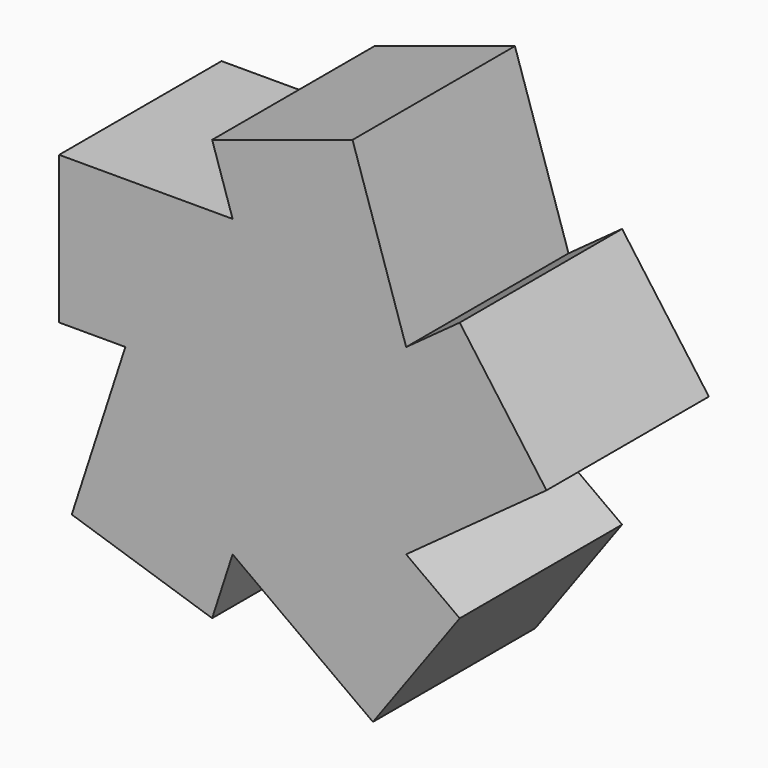
from build123d import *

# Parameters (mm, degrees)
F0_W     = 60
F0_H     = 55
F1_DEPTH = 40
F2_COUNT = 5


with BuildPart() as f1:
    # F0 (on Top) → F1 (new body)
    with BuildSketch(Plane.XY):
        with Locations((-30, 27.5)):
            Rectangle(F0_W, F0_H)
    extrude(amount=F1_DEPTH)

    # F2: F1 ×5 about axis
    f2_axis = Axis((0, 27.5, 0), (0, -1, 0))


with BuildPart() as f1_1:
    add(f1.part)
    for i in range(1, F2_COUNT):
        add(f1.part.rotate(f2_axis, i * 360 / F2_COUNT))


solid = f1_1.part
